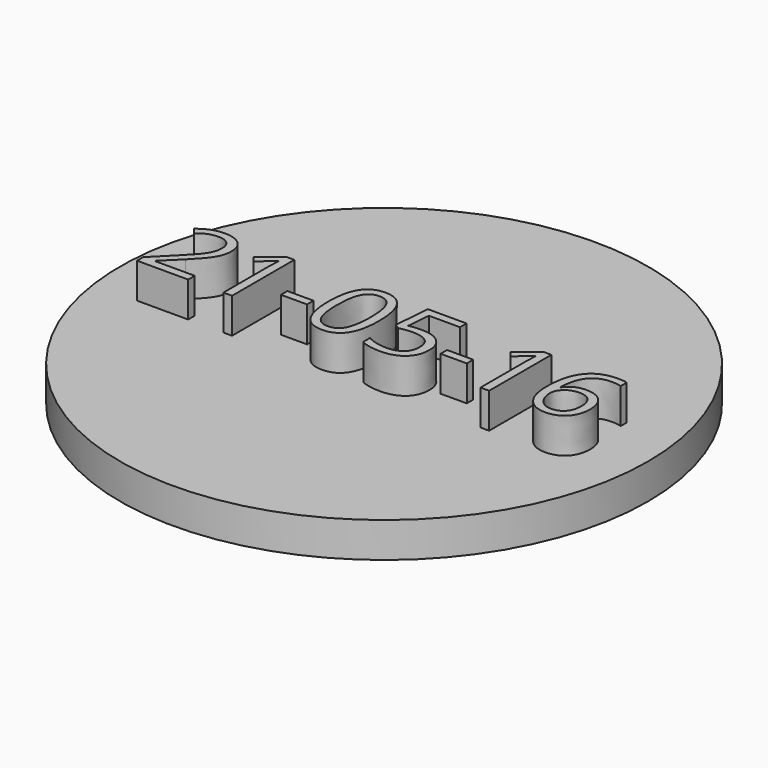
from build123d import *

# Parameters (mm, degrees)
F0_R         = 15
F1_DEPTH     = 2
F2_TEXT_SIZE = 6.1945134671
F3_DEPTH     = 2


# Not quite as in the source:
# - Text() gives the source's letters only with a copy of the font that has no kerning and outlines rounded to 1/6400 em; it was checked with that copy


with BuildPart() as f1:
    # F0 (on Top) → F1 (new body)
    with BuildSketch(Plane.XY):
        Circle(F0_R)
    extrude(amount=F1_DEPTH)

    # F2 (on face) → F3 (join)
    with BuildSketch(Plane.XY.offset(2)):
        with Locations((-12.6672960939, -2.0964924322)):
            Text('21-05-16', F2_TEXT_SIZE, font='Open Sans', text_align=(TextAlign.LEFT, TextAlign.BOTTOM))
    extrude(amount=F3_DEPTH)


solid = f1.part
